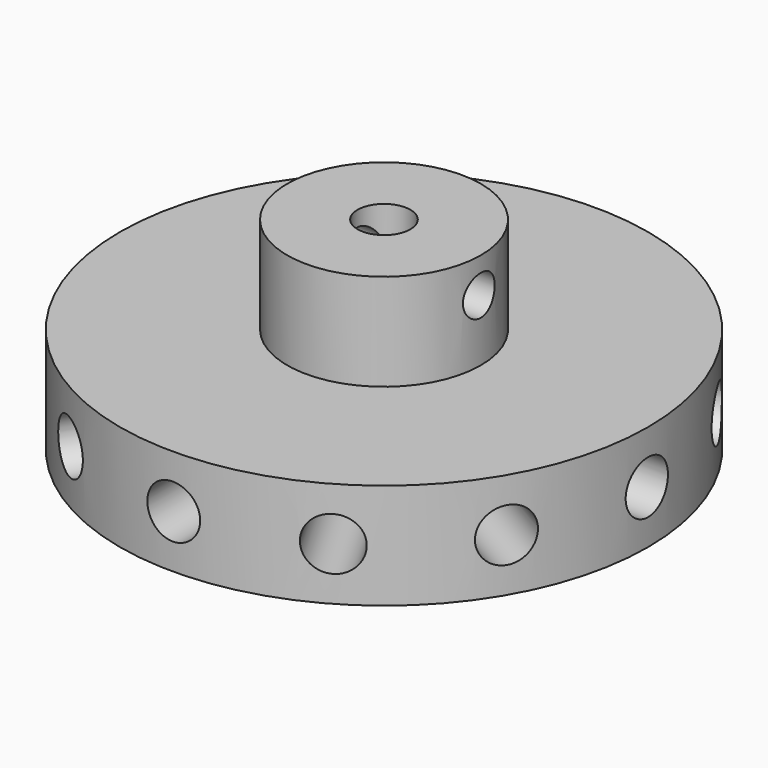
from build123d import *
from build123d import SkipClean  # not in build123d's __all__

# Parameters (mm, degrees)
F4_R              = 30
F5_DEPTH          = 12
F6_R              = 11
F7_DEPTH          = 11
F9_D              = 6
F10_R             = 2.25
F11_DEPTH         = 50
F14_R             = 3
F15_DEPTH         = 15
F15_COPIES_COUNT  = 3
F15_COPIES_ANGLE  = 120
F15_COPIES1_COUNT = 3
F15_COPIES1_ANGLE = 300
F17_R             = 3
F18_DEPTH         = 15
F20_R             = 3
F21_DEPTH         = 15
F23_R             = 3
F24_DEPTH         = 15
F30_R             = 3
F31_DEPTH         = 15
F33_R             = 3
F34_DEPTH         = 15
F36_R             = 3
F37_DEPTH         = 15
F39_R             = 3
F40_DEPTH         = 15
F42_R             = 3
F43_DEPTH         = 15
F45_R             = 3
F46_DEPTH         = 15
F48_R             = 3
F49_DEPTH         = 15
F51_R             = 3
F52_DEPTH         = 15


# Not quite as in the source:
# - a pattern or mirror of a feature is missing from the dataset's text; its kind, count and spacing are read off the source's solid


with BuildPart() as f5:
    # F4 (on Top) → F5 (new body)
    with BuildSketch(Plane.XY):
        Circle(F4_R)
    extrude(amount=F5_DEPTH)

    # F6 (on face) → F7 (join)
    with BuildSketch(Plane.XY.offset(12)):
        Circle(F6_R)
    extrude(amount=F7_DEPTH)

    # F9 (through all)
    with Locations(Plane.XY.offset(23)):
        with Locations((0, 0)):
            Hole(F9_D / 2)

    # F10 (on Right) → F11 (cut, symmetric)
    with BuildSketch(Plane.YZ):
        with Locations((0, 19)):
            Circle(F10_R)
    extrude(amount=F11_DEPTH, both=True, mode=Mode.SUBTRACT)

    # F14 (on offset) → F15 (cut)
    with BuildSketch(Plane.XZ.offset(30)):
        with Locations((0, 6)):
            Circle(F14_R)
    f15 = extrude(amount=-F15_DEPTH, mode=Mode.SUBTRACT)

    # F15_copies: F15 ×3 about axis
    f15_copies_axis = Axis((0, 0, 0), (0, 0, 1))
    for i in range(1, F15_COPIES_COUNT):
        add(f15.rotate(f15_copies_axis, i * F15_COPIES_ANGLE / (F15_COPIES_COUNT - 1)), clean=False, mode=Mode.SUBTRACT)

    # F15_copies1: F15 ×3 about axis
    f15_copies1_axis = Axis((0, 0, 0), (0, 0, 1))
    for i in range(1, F15_COPIES1_COUNT):
        add(f15.rotate(f15_copies1_axis, i * F15_COPIES1_ANGLE / (F15_COPIES1_COUNT - 1)), clean=False, mode=Mode.SUBTRACT)

    # F15_copies2: F15 across plane
    add(f15.mirror(Plane(origin=(0, 0, 0), x_dir=(-0.2588190451, -0.9659258263, 0), z_dir=(-0.9659258263, 0.2588190451, 0))), clean=False, mode=Mode.SUBTRACT)

    # F15_copies3: F15 across plane
    add(f15.mirror(Plane(origin=(0, 0, 0), x_dir=(0.8660254038, 0.5, 0), z_dir=(-0.5, 0.8660254038, 0))), clean=False, mode=Mode.SUBTRACT)

    # F17 (on offset) → F18 (cut)
    with BuildSketch(Plane.XZ.offset(-30)):
        with Locations((0, 6)):
            Circle(F17_R)
    extrude(amount=F18_DEPTH, mode=Mode.SUBTRACT)

    # F20 (on offset) → F21 (cut)
    with BuildSketch(Plane.YZ.offset(30)):
        with Locations((0, 6)):
            Circle(F20_R)
    extrude(amount=-F21_DEPTH, mode=Mode.SUBTRACT)

    # F23 (on offset) → F24 (join)
    with BuildSketch(Plane.YZ.offset(-30)):
        with Locations((0, 6)):
            Circle(F23_R)
    with SkipClean():  # cleaning this boolean's faces spoils the solid; the shape is the same uncleaned
        extrude(amount=F24_DEPTH)

    # F30 (on face) → F31 (cut)
    with BuildSketch(Plane(origin=(25.9807621135, -15, 0), x_dir=(-0.5, -0.8660254038, 0), z_dir=(-0.8660254038, 0.5, 0))):
        with Locations((0, 6)):
            Circle(F30_R)
    with SkipClean():  # cleaning this boolean's faces spoils the solid; the shape is the same uncleaned
        extrude(amount=-F31_DEPTH, mode=Mode.SUBTRACT)

    # F33 (on face) → F34 (cut)
    with BuildSketch(Plane(origin=(-25.9807621135, 15, 0), x_dir=(-0.5, -0.8660254038, 0), z_dir=(-0.8660254038, 0.5, 0))):
        with Locations((0, 6)):
            Circle(F33_R)
    with SkipClean():  # cleaning this boolean's faces spoils the solid; the shape is the same uncleaned
        extrude(amount=F34_DEPTH, mode=Mode.SUBTRACT)

    # F36 (on face) → F37 (cut)
    with BuildSketch(Plane(origin=(-25.9807621135, -15, 0), x_dir=(0.5, -0.8660254038, 0), z_dir=(-0.8660254038, -0.5, 0))):
        with Locations((0, 6)):
            Circle(F36_R)
    with SkipClean():  # cleaning this boolean's faces spoils the solid; the shape is the same uncleaned
        extrude(amount=F37_DEPTH, mode=Mode.SUBTRACT)

    # F39 (on face) → F40 (cut)
    with BuildSketch(Plane(origin=(15, -25.9807621135, 0), x_dir=(-0.8660254038, -0.5, 0), z_dir=(-0.5, 0.8660254038, 0))):
        with Locations((0, 6)):
            Circle(F39_R)
    with SkipClean():  # cleaning this boolean's faces spoils the solid; the shape is the same uncleaned
        extrude(amount=F40_DEPTH, mode=Mode.SUBTRACT)

    # F42 (on face) → F43 (cut)
    with BuildSketch(Plane(origin=(-15, -25.9807621135, 0), x_dir=(0.8660254038, -0.5, 0), z_dir=(-0.5, -0.8660254038, 0))):
        with Locations((0, 6)):
            Circle(F42_R)
    with SkipClean():  # cleaning this boolean's faces spoils the solid; the shape is the same uncleaned
        extrude(amount=F43_DEPTH, mode=Mode.SUBTRACT)

    # F45 (on face) → F46 (cut)
    with BuildSketch(Plane(origin=(15, 25.9807621135, 0), x_dir=(0.8660254038, -0.5, 0), z_dir=(-0.5, -0.8660254038, 0))):
        with Locations((0, 6)):
            Circle(F45_R)
    with SkipClean():  # cleaning this boolean's faces spoils the solid; the shape is the same uncleaned
        extrude(amount=-F46_DEPTH, mode=Mode.SUBTRACT)

    # F48 (on face) → F49 (cut)
    with BuildSketch(Plane(origin=(25.9807621135, 15, 0), x_dir=(0.5, -0.8660254038, 0), z_dir=(-0.8660254038, -0.5, 0))):
        with Locations((0, 6)):
            Circle(F48_R)
    with SkipClean():  # cleaning this boolean's faces spoils the solid; the shape is the same uncleaned
        extrude(amount=-F49_DEPTH, mode=Mode.SUBTRACT)

    # F51 (on face) → F52 (join)
    with BuildSketch(Plane(origin=(-15, 25.9807621135, 0), x_dir=(-0.8660254038, -0.5, 0), z_dir=(-0.5, 0.8660254038, 0))):
        with Locations((0, 6)):
            Circle(F51_R)
    with SkipClean():  # cleaning this boolean's faces spoils the solid; the shape is the same uncleaned
        extrude(amount=-F52_DEPTH)


solid = f5.part
